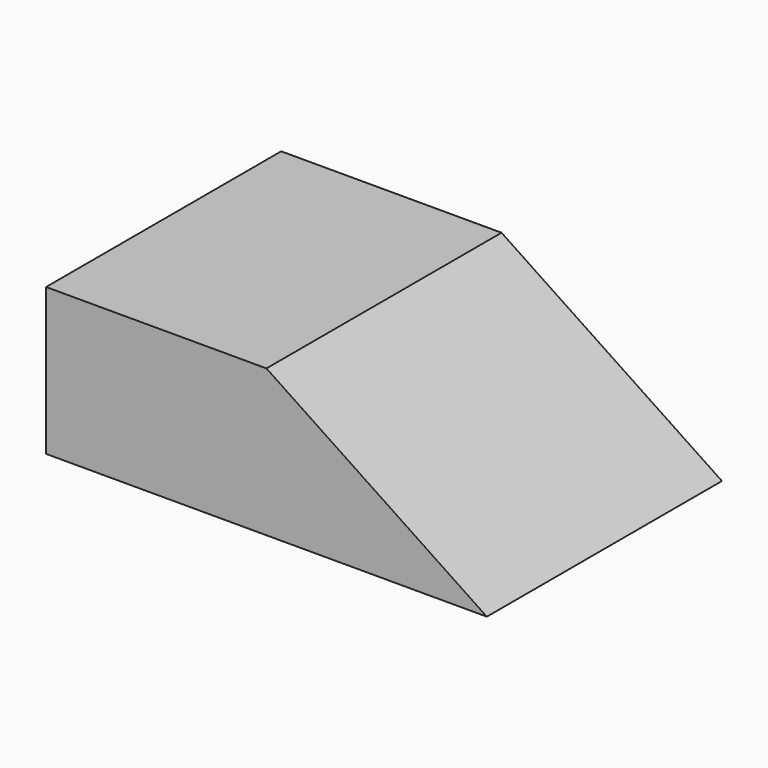
from build123d import *

# Parameters (mm, degrees)
F0_W     = 1828.8
F0_H     = 1219.2
F1_DEPTH = 1219.2


# Not quite as in the source:
# - a feature names something its author has since deleted; it is built from what else it names


with BuildPart() as f1:
    # F0 (on Front) → F1 (new body, symmetric)
    with BuildSketch(Plane.XZ):
        with Locations((914.4, 609.6)):
            Rectangle(F0_W, F0_H)
        Polygon((1828.8, 1219.2), (1828.8, 0), (3657.6, 0), align=None)
    extrude(amount=F1_DEPTH, both=True)


solid = f1.part
